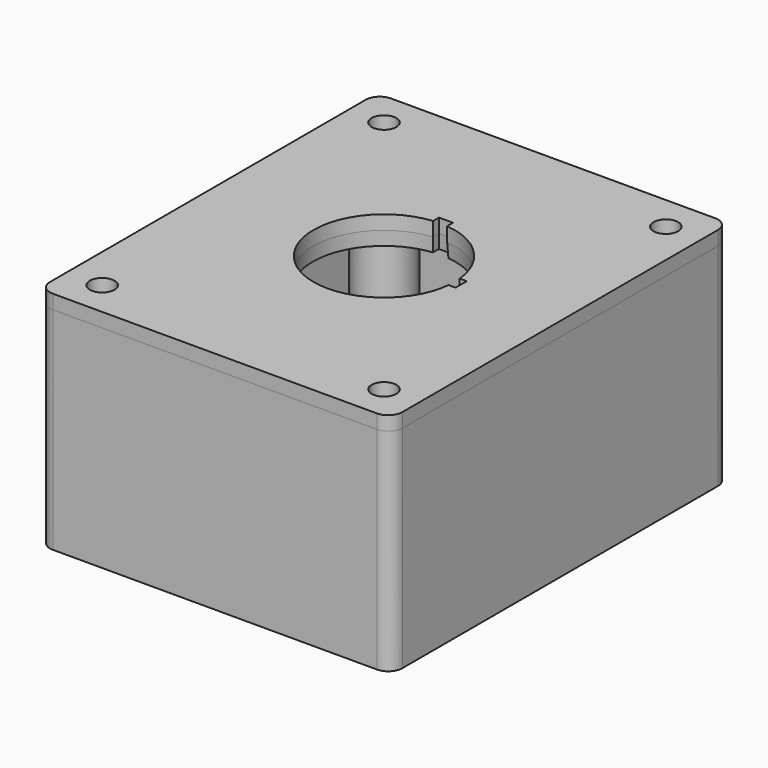
from build123d import *

# Parameters (mm, degrees)
F0_W     = 50
F0_H     = 60
F0_R     = 1.45
F0_R_2   = 2.5
F0_R_3   = 10
F1_DEPTH = 30
F2_T     = -2.5
F4_DEPTH = 2
F4_TAPER = 3
F3_W     = 50
F3_H     = 60
F3_R     = 1.75
F5_DEPTH = 2
F6_R     = 2
F6_2_R   = 2


with BuildPart() as f1:
    # F0 (on Top) → F1 (new body)
    with BuildSketch(Plane.XY):
        Rectangle(F0_W, F0_H)
        with Locations((-20, -25)):
            Circle(F0_R, mode=Mode.SUBTRACT)
        with Locations((0, -20)):
            Circle(F0_R_2, mode=Mode.SUBTRACT)
        with Locations((20, -25)):
            Circle(F0_R, mode=Mode.SUBTRACT)
        with Locations((-20, 25)):
            Circle(F0_R, mode=Mode.SUBTRACT)
        Circle(F0_R_3, mode=Mode.SUBTRACT)
        with Locations((0, 20)):
            Circle(F0_R_2, mode=Mode.SUBTRACT)
        with Locations((20, 25)):
            Circle(F0_R, mode=Mode.SUBTRACT)
    extrude(amount=F1_DEPTH)

    # F2
    f2_openings = [f1.faces().sort_by_distance(p)[0] for p in [
        (-10, 0, 15),
        (0, -29.218975, 30),
        (-2.5, 20, 15),
        (-2.5, -20, 15),
    ]]
    offset(amount=F2_T, openings=f2_openings)

    # F6
    f6_edges = [f1.edges().sort_by_distance(p)[0] for p in [
        (25, 30, 15),
        (25, -30, 15),
        (-25, 30, 15),
        (-25, -30, 15),
    ]]
    fillet(f6_edges, radius=F6_R)


with BuildPart() as f4:
    # F3 (on face) → F4 (new body)
    with BuildSketch(Plane.XY.offset(30)):
        with BuildLine():
            ThreePointArc((-22.1, -21.1904724702), (-16.9240855018, -21.9240855018), (-16.1904724702, -27.1))
            Line((-16.1904724702, -27.1), (16.1904724702, -27.1))
            ThreePointArc((16.1904724702, -27.1), (16.9240855018, -21.9240855018), (22.1, -21.1904724702))
            Line((22.1, -21.1904724702), (22.1, 21.1904724702))
            ThreePointArc((22.1, 21.1904724702), (16.9240855018, 21.9240855018), (16.1904724702, 27.1))
            Line((16.1904724702, 27.1), (-16.1904724702, 27.1))
            ThreePointArc((-16.1904724702, 27.1), (-16.9240855018, 21.9240855018), (-22.1, 21.1904724702))
            Line((-22.1, 21.1904724702), (-22.1, -21.1904724702))
        make_face()
        with BuildLine():
            ThreePointArc((9.9498743711, -1), (-7.0710678119, -7.0710678119), (-1, 9.9498743711))
            Line((-1, 9.9498743711), (-1, 11))
            Line((-1, 11), (1, 11))
            Line((1, 11), (1, 9.9498743711))
            ThreePointArc((1, 9.9498743711), (7.0710678119, 7.0710678119), (9.9498743711, 1))
            Line((9.9498743711, 1), (10.9498743711, 1))
            Line((10.9498743711, 1), (10.9498743711, -1))
            Line((10.9498743711, -1), (9.9498743711, -1))
        make_face(mode=Mode.SUBTRACT)
    extrude(amount=-F4_DEPTH, taper=F4_TAPER)

    # F3 (on face) → F5 (join)
    with BuildSketch(Plane.XY.offset(30)):
        Rectangle(F3_W, F3_H)
        with Locations((-20, -25)):
            Circle(F3_R, mode=Mode.SUBTRACT)
        with Locations((20, -25)):
            Circle(F3_R, mode=Mode.SUBTRACT)
        with Locations((-20, 25)):
            Circle(F3_R, mode=Mode.SUBTRACT)
        with BuildLine():
            ThreePointArc((-16.05, -25), (-18.3077381999, -21.4308614485), (-22.5, -21.9418142633))
            Line((-22.5, -21.9418142633), (-22.5, 21.9418142633))
            ThreePointArc((-22.5, 21.9418142633), (-18.3077381999, 21.4308614485), (-16.05, 25))
            ThreePointArc((-16.05, 25), (-16.2796281328, 26.3271522784), (-16.9418142633, 27.5))
            Line((-16.9418142633, 27.5), (16.9418142633, 27.5))
            ThreePointArc((16.9418142633, 27.5), (17.2069282143, 22.2069282143), (22.5, 21.9418142633))
            Line((22.5, 21.9418142633), (22.5, -21.9418142633))
            ThreePointArc((22.5, -21.9418142633), (17.2069282143, -22.2069282143), (16.9418142633, -27.5))
            Line((16.9418142633, -27.5), (-16.9418142633, -27.5))
            ThreePointArc((-16.9418142633, -27.5), (-16.2796281328, -26.3271522784), (-16.05, -25))
        make_face(mode=Mode.SUBTRACT)
        with Locations((20, 25)):
            Circle(F3_R, mode=Mode.SUBTRACT)
        with BuildLine():
            Line((-22.5, 21.9418142633), (-22.5, -21.9418142633))
            ThreePointArc((-22.5, -21.9418142633), (-18.3077381999, -21.4308614485), (-16.05, -25))
            ThreePointArc((-16.05, -25), (-16.2796281328, -26.3271522784), (-16.9418142633, -27.5))
            Line((-16.9418142633, -27.5), (16.9418142633, -27.5))
            ThreePointArc((16.9418142633, -27.5), (17.2069282143, -22.2069282143), (22.5, -21.9418142633))
            Line((22.5, -21.9418142633), (22.5, 21.9418142633))
            ThreePointArc((22.5, 21.9418142633), (17.2069282143, 22.2069282143), (16.9418142633, 27.5))
            Line((16.9418142633, 27.5), (-16.9418142633, 27.5))
            ThreePointArc((-16.9418142633, 27.5), (-16.2796281328, 26.3271522784), (-16.05, 25))
            ThreePointArc((-16.05, 25), (-18.3077381999, 21.4308614485), (-22.5, 21.9418142633))
        make_face()
        with BuildLine():
            Line((16.1904724702, -27.1), (-16.1904724702, -27.1))
            ThreePointArc((-16.1904724702, -27.1), (-16.9240855018, -21.9240855018), (-22.1, -21.1904724702))
            Line((-22.1, -21.1904724702), (-22.1, 21.1904724702))
            ThreePointArc((-22.1, 21.1904724702), (-16.9240855018, 21.9240855018), (-16.1904724702, 27.1))
            Line((-16.1904724702, 27.1), (16.1904724702, 27.1))
            ThreePointArc((16.1904724702, 27.1), (16.9240855018, 21.9240855018), (22.1, 21.1904724702))
            Line((22.1, 21.1904724702), (22.1, -21.1904724702))
            ThreePointArc((22.1, -21.1904724702), (16.9240855018, -21.9240855018), (16.1904724702, -27.1))
        make_face(mode=Mode.SUBTRACT)
        with BuildLine():
            ThreePointArc((-22.1, -21.1904724702), (-16.9240855018, -21.9240855018), (-16.1904724702, -27.1))
            Line((-16.1904724702, -27.1), (16.1904724702, -27.1))
            ThreePointArc((16.1904724702, -27.1), (16.9240855018, -21.9240855018), (22.1, -21.1904724702))
            Line((22.1, -21.1904724702), (22.1, 21.1904724702))
            ThreePointArc((22.1, 21.1904724702), (16.9240855018, 21.9240855018), (16.1904724702, 27.1))
            Line((16.1904724702, 27.1), (-16.1904724702, 27.1))
            ThreePointArc((-16.1904724702, 27.1), (-16.9240855018, 21.9240855018), (-22.1, 21.1904724702))
            Line((-22.1, 21.1904724702), (-22.1, -21.1904724702))
        make_face()
        with BuildLine():
            ThreePointArc((9.9498743711, -1), (-7.0710678119, -7.0710678119), (-1, 9.9498743711))
            Line((-1, 9.9498743711), (-1, 11))
            Line((-1, 11), (1, 11))
            Line((1, 11), (1, 9.9498743711))
            ThreePointArc((1, 9.9498743711), (7.0710678119, 7.0710678119), (9.9498743711, 1))
            Line((9.9498743711, 1), (10.9498743711, 1))
            Line((10.9498743711, 1), (10.9498743711, -1))
            Line((10.9498743711, -1), (9.9498743711, -1))
        make_face(mode=Mode.SUBTRACT)
    extrude(amount=F5_DEPTH)

    # F6#2
    f6_2_edges = [f4.edges().sort_by_distance(p)[0] for p in [
        (25, 30, 31),
        (25, -30, 31),
        (-25, 30, 31),
        (-25, -30, 31),
    ]]
    fillet(f6_2_edges, radius=F6_2_R)


solid = Compound([f1.part, f4.part])
